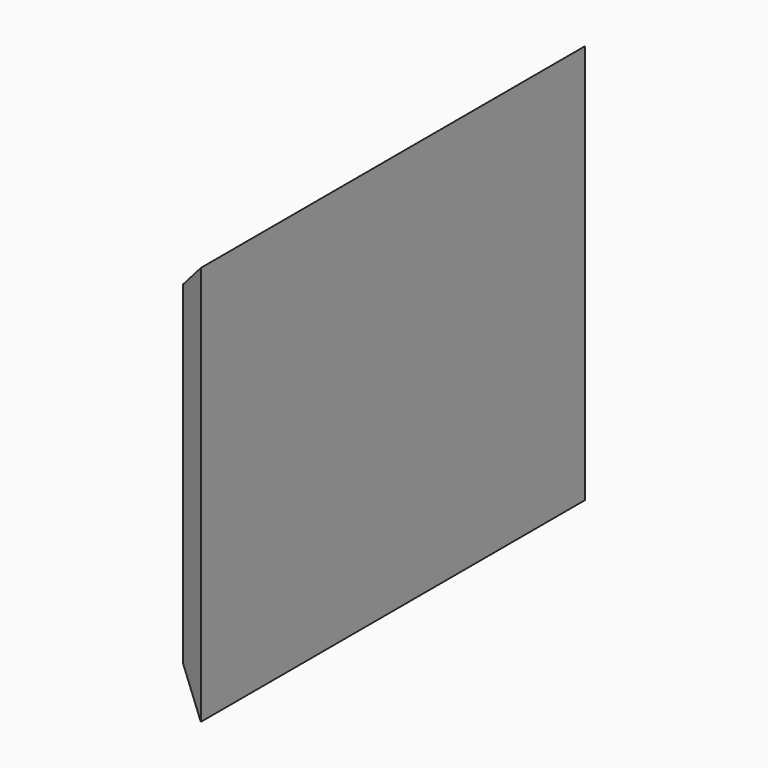
from build123d import *

# Parameters (mm, degrees)
F0_W     = 285.75
F0_H     = 228.6
F1_DEPTH = 19.05
F3_DEPTH = 228.601
F4_SIZE  = 19.04999


# Not quite as in the source:
# - a fillet or chamfer is up to 0.001 mm smaller than in the source, because OpenCascade refuses the exact size


with BuildPart() as f1:
    # F0 (on Right) → F1 (new body)
    with BuildSketch(Plane.YZ):
        Rectangle(F0_W, F0_H)
    extrude(amount=F1_DEPTH)

    # F2 (on face) → F3 (cut, through all)
    with BuildSketch(Plane.XY.offset(114.3)):
        Polygon((0, -142.875), (19.05, -142.875), (0, -131.8764773719), align=None)
        Polygon((19.05, 142.875), (0, 142.875), (19.05, 131.8764773719), align=None)
    extrude(amount=-F3_DEPTH, mode=Mode.SUBTRACT)

    # F4 (size 19.05 in the source; OpenCascade refuses exactly that, so slightly less here)
    f4_edges = [f1.edges().sort_by_distance(p)[0] for p in [
        (0, 5.499261, 114.3),
        (0, 5.499261, -114.3),
    ]]
    chamfer(f4_edges, length=F4_SIZE)


solid = f1.part
